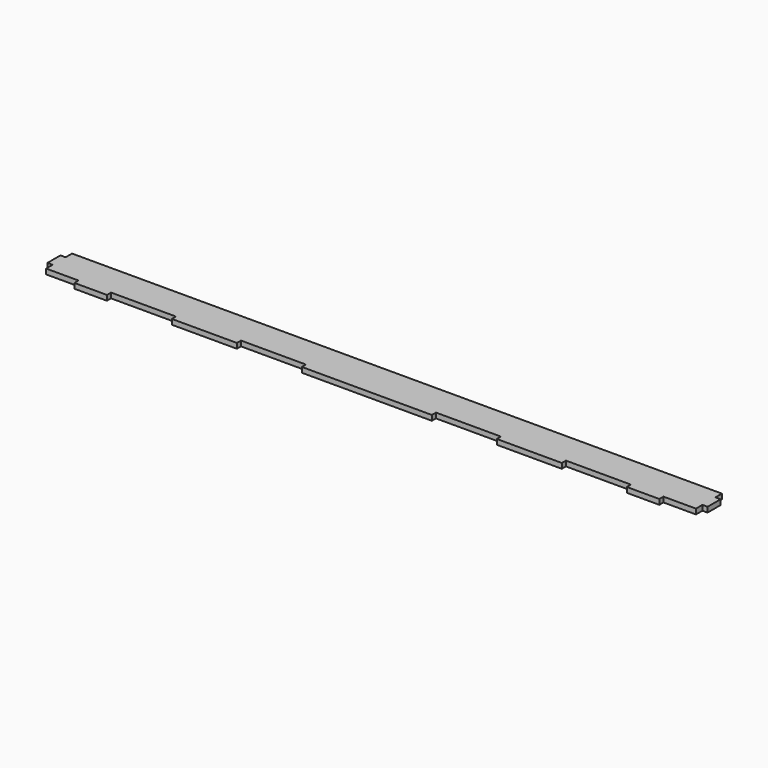
from build123d import *

# Parameters (mm, degrees)
F0_W     = 10
F0_H     = 1.5875
F0_W_2   = 1.5875
F0_H_2   = 5
F0_W_3   = 20
F0_W_4   = 40
F1_DEPTH = 1.5875


# Not quite as in the source:
# - a length typed as a fraction of an inch, garbled in the dataset ("3 / 203.2 mm" for 3/8 in), is restored


with BuildPart() as f1:
    # F0 (on Top) → F1 (new body)
    with BuildSketch(Plane.XY):
        Polygon((-100, -2.5), (-100, -5), (-90, -5), (-80, -5), (-60, -5), (-40, -5), (-20, -5), (20, -5), (40, -5), (60, -5), (80, -5), (90, -5), (100, -5), (100, -2.5), (100, 2.5), (100, 5), (-100, 5), (-100, 2.5), align=None)
        with Locations((-85, -5.79375)):
            Rectangle(F0_W, F0_H)
        with Locations((-100.79375, 0)):
            Rectangle(F0_W_2, F0_H_2)
        with Locations((-50, -5.79375)):
            Rectangle(F0_W_3, F0_H)
        with Locations((0, -5.79375)):
            Rectangle(F0_W_4, F0_H)
        with Locations((100.79375, 0)):
            Rectangle(F0_W_2, F0_H_2)
        with Locations((50, -5.79375)):
            Rectangle(F0_W_3, F0_H)
        with Locations((85, -5.79375)):
            Rectangle(F0_W, F0_H)
    extrude(amount=F1_DEPTH)


solid = f1.part
